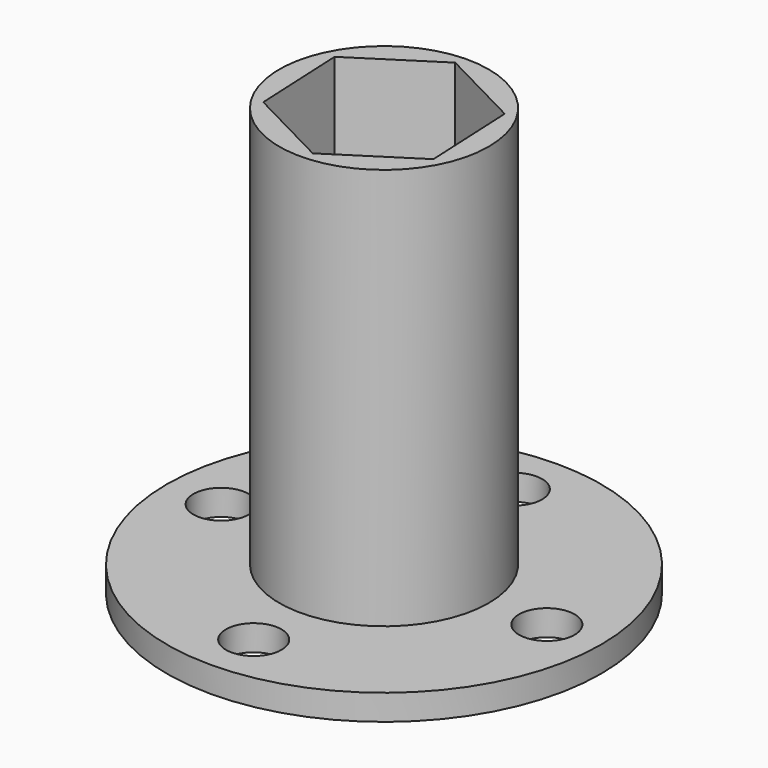
from build123d import *

# Parameters (mm, degrees)
F1_R     = 12.25
F2_DEPTH = 47
F3_DEPTH = 45
F4_R     = 7.5
F5_DEPTH = 25
F6_R     = 25.4
F6_R_2   = 3.25
F6_R_3   = 12.25
F6_R_4   = 7.5
F7_DEPTH = 3


with BuildPart() as f2:
    # F1 (on Top) → F2 (new body)
    with BuildSketch(Plane.XY):
        Circle(F1_R)
    extrude(amount=-F2_DEPTH)

    # F0 (on Top) → F3 (cut)
    with BuildSketch(Plane.XY):
        Polygon((-0.5242376146, 11.0727221099), (-9.8513774435, 5.0823579631), (-9.327139829, -5.9903641468), (0.5242376146, -11.0727221099), (9.8513774435, -5.0823579631), (9.327139829, 5.9903641468), align=None)
    extrude(amount=-F3_DEPTH, mode=Mode.SUBTRACT)

    # F4 (on face) → F5 (cut)
    with BuildSketch(Plane(origin=(0, 0, -47), x_dir=(1, 0, 0), z_dir=(0, 0, -1))):
        Circle(F4_R)
    extrude(amount=-F5_DEPTH, mode=Mode.SUBTRACT)


with BuildPart() as f7:
    # F6 (on face) → F7 (new body)
    with BuildSketch(Plane(origin=(0, 0, -47), x_dir=(1, 0, 0), z_dir=(0, 0, -1))):
        Circle(F6_R)
        with Locations((0, -19.05)):
            Circle(F6_R_2, mode=Mode.SUBTRACT)
        with Locations((-19.05, 0)):
            Circle(F6_R_2, mode=Mode.SUBTRACT)
        Circle(F6_R_3, mode=Mode.SUBTRACT)
        with Locations((19.05, 0)):
            Circle(F6_R_2, mode=Mode.SUBTRACT)
        with Locations((0, 19.05)):
            Circle(F6_R_2, mode=Mode.SUBTRACT)
        Circle(F6_R_3)
        Circle(F6_R_4, mode=Mode.SUBTRACT)
    extrude(amount=F7_DEPTH)


solid = Compound([f2.part, f7.part])
